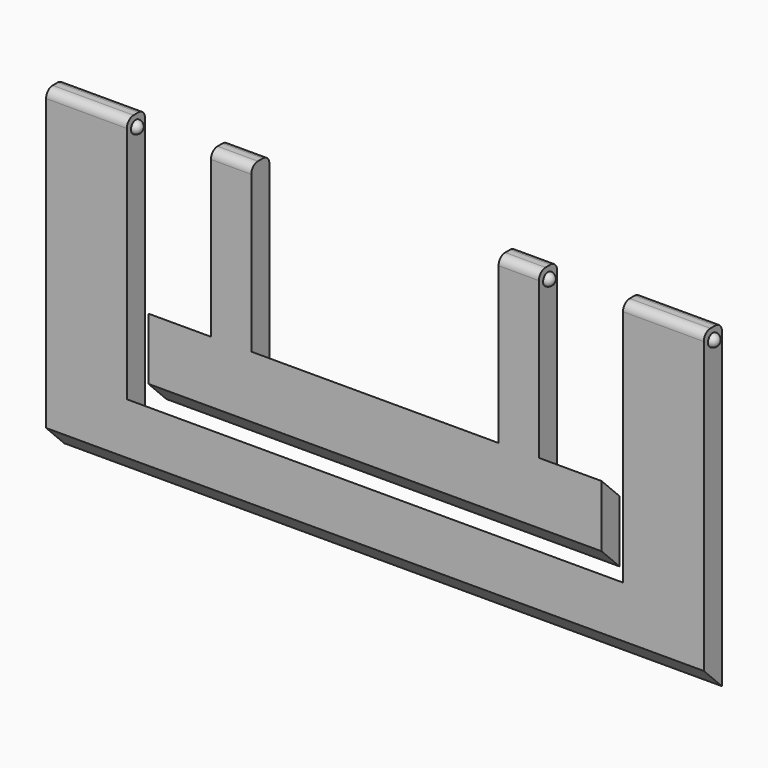
from build123d import *

# Parameters (mm, degrees)
F1_DEPTH       = 79.8
F1_DEPTH_BACK  = 79.8
F2_DEPTH       = 60.2
F2_DEPTH_BACK  = 60.2
F3_DEPTH       = 55
F3_DEPTH_BACK  = 55
F4_DEPTH       = 39.8
F4_DEPTH_BACK  = 39.8
F5_DEPTH       = 20.2
F5_DEPTH_BACK  = 20.2
F6_R           = 1.5
F7_DEPTH       = 1.5
F7_DEPTH_BACK  = 21.1
F8_R           = 1.49999
F9_R           = 1.5
F10_DEPTH      = 1.5
F10_DEPTH_BACK = 21.1
F11_R          = 1.49999
F12_R          = 1.5
F13_DEPTH      = 1.5
F13_DEPTH_BACK = 21.1
F14_R          = 1.49999
F15_R          = 1.5
F16_DEPTH      = 1.5
F16_DEPTH_BACK = 21.1
F17_R          = 1.49999
F18_DEPTH      = 30
F18_DEPTH_BACK = 30


# Not quite as in the source:
# - a fillet or chamfer is up to 0.001 mm smaller than in the source, because OpenCascade refuses the exact size


with BuildPart() as f1:
    # F0 (on Right) → F1 (new body, two sides)
    with BuildSketch(Plane.YZ) as f1_sk:
        with BuildLine():
            Line((-5.401472277, 44.6310500277), (-5.401472277, 79.9993566108))
            Line((-5.401472277, 79.9993566108), (-5.401472277, 88))
            ThreePointArc((-5.401472277, 88), (-5.9872587146, 89.4142135624), (-7.401472277, 90))
            Line((-7.401472277, 90), (-8.901472277, 90))
            ThreePointArc((-8.901472277, 90), (-10.3156858394, 89.4142135624), (-10.901472277, 88))
            Line((-10.901472277, 88), (-10.901472277, 80))
            Line((-10.901472277, 80), (-10.901472277, 50.1310500277))
            Line((-10.901472277, 50.1310500277), (-5.401472277, 44.6310500277))
        make_face()
        Polygon((-5.401472277, 29.6310500277), (-5.401472277, 44.6310500277), (-10.901472277, 50.1310500277), (-10.901472277, 35.1310500277), align=None)
        Polygon((-5.401472277, 24.6310500277), (-5.401472277, 29.6310500277), (-10.901472277, 35.1310500277), (-10.901472277, 30.1310500277), align=None)
        Polygon((-5.401472277, 18.0382234147), (-5.401472277, 24.6310500277), (-10.901472277, 30.1310500277), (-10.901472277, 17.6310500277), (-5.401472277, 12.1310500277), align=None)
    extrude(amount=F1_DEPTH)
    extrude(f1_sk.sketch, amount=-F1_DEPTH_BACK)

    # F0 (on Right) → F2 (cut, two sides)
    with BuildSketch(Plane.YZ) as f2_sk:
        Polygon((-5.401472277, 24.6310500277), (-5.401472277, 29.6310500277), (-10.901472277, 35.1310500277), (-10.901472277, 30.1310500277), align=None)
        Polygon((-5.401472277, 29.6310500277), (-5.401472277, 44.6310500277), (-10.901472277, 50.1310500277), (-10.901472277, 35.1310500277), align=None)
        with BuildLine():
            Line((-5.401472277, 44.6310500277), (-5.401472277, 79.9993566108))
            Line((-5.401472277, 79.9993566108), (-5.401472277, 88))
            ThreePointArc((-5.401472277, 88), (-5.9872587146, 89.4142135624), (-7.401472277, 90))
            Line((-7.401472277, 90), (-8.901472277, 90))
            ThreePointArc((-8.901472277, 90), (-10.3156858394, 89.4142135624), (-10.901472277, 88))
            Line((-10.901472277, 88), (-10.901472277, 80))
            Line((-10.901472277, 80), (-10.901472277, 50.1310500277))
            Line((-10.901472277, 50.1310500277), (-5.401472277, 44.6310500277))
        make_face()
    extrude(amount=F2_DEPTH, mode=Mode.SUBTRACT)
    extrude(f2_sk.sketch, amount=-F2_DEPTH_BACK, mode=Mode.SUBTRACT)

    # F6 (on face) → F7 (join, two sides)
    with BuildSketch(Plane(origin=(-79.8, 0, 0), x_dir=(0, -1, 0), z_dir=(-1, 0, 0))) as f7_sk:
        with Locations((8.151472277, 87.25)):
            Circle(F6_R)
    extrude(amount=F7_DEPTH)
    extrude(f7_sk.sketch, amount=-F7_DEPTH_BACK)

    # F8 (radius 1.5 in the source; OpenCascade refuses exactly that, so slightly less here)
    f8_edges = [f1.edges().sort_by_distance(p)[0] for p in [
        (-81.3, -6.651472, 87.25),
        (-58.7, -6.651472, 87.25),
    ]]
    fillet(f8_edges, radius=F8_R)

    # F15 (on face) → F16 (join, two sides)
    with BuildSketch(Plane(origin=(60.2, 0, 0), x_dir=(0, -1, 0), z_dir=(-1, 0, 0))) as f16_sk:
        with Locations((8.151472277, 87.25)):
            Circle(F15_R)
    extrude(amount=F16_DEPTH)
    extrude(f16_sk.sketch, amount=-F16_DEPTH_BACK)

    # F17 (radius 1.5 in the source; OpenCascade refuses exactly that, so slightly less here)
    f17_edges = [f1.edges().sort_by_distance(p)[0] for p in [
        (58.7, -6.651472, 87.25),
        (81.3, -6.651472, 87.25),
    ]]
    fillet(f17_edges, radius=F17_R)


with BuildPart() as f3:
    # F0 (on Right) → F3 (new body, two sides)
    with BuildSketch(Plane.YZ) as f3_sk:
        Polygon((-5.401472277, 29.6310500277), (-5.401472277, 44.6310500277), (-10.901472277, 50.1310500277), (-10.901472277, 35.1310500277), align=None)
    extrude(amount=F3_DEPTH)
    extrude(f3_sk.sketch, amount=-F3_DEPTH_BACK)

    # F0 (on Right) → F4 (join, two sides)
    with BuildSketch(Plane.YZ) as f4_sk:
        with BuildLine():
            Line((-5.401472277, 44.6310500277), (-5.401472277, 79.9993566108))
            Line((-5.401472277, 79.9993566108), (-5.401472277, 88))
            ThreePointArc((-5.401472277, 88), (-5.9872587146, 89.4142135624), (-7.401472277, 90))
            Line((-7.401472277, 90), (-8.901472277, 90))
            ThreePointArc((-8.901472277, 90), (-10.3156858394, 89.4142135624), (-10.901472277, 88))
            Line((-10.901472277, 88), (-10.901472277, 80))
            Line((-10.901472277, 80), (-10.901472277, 50.1310500277))
            Line((-10.901472277, 50.1310500277), (-5.401472277, 44.6310500277))
        make_face()
    extrude(amount=F4_DEPTH)
    extrude(f4_sk.sketch, amount=-F4_DEPTH_BACK)

    # F0 (on Right) → F5 (cut, two sides)
    with BuildSketch(Plane.YZ) as f5_sk:
        with BuildLine():
            Line((-5.401472277, 44.6310500277), (-5.401472277, 79.9993566108))
            Line((-5.401472277, 79.9993566108), (-5.401472277, 88))
            ThreePointArc((-5.401472277, 88), (-5.9872587146, 89.4142135624), (-7.401472277, 90))
            Line((-7.401472277, 90), (-8.901472277, 90))
            ThreePointArc((-8.901472277, 90), (-10.3156858394, 89.4142135624), (-10.901472277, 88))
            Line((-10.901472277, 88), (-10.901472277, 80))
            Line((-10.901472277, 80), (-10.901472277, 50.1310500277))
            Line((-10.901472277, 50.1310500277), (-5.401472277, 44.6310500277))
        make_face()
    extrude(amount=F5_DEPTH, mode=Mode.SUBTRACT)
    extrude(f5_sk.sketch, amount=-F5_DEPTH_BACK, mode=Mode.SUBTRACT)

    # F9 (on face) → F10 (join, two sides)
    with BuildSketch(Plane(origin=(-39.8, 0, 0), x_dir=(0, -1, 0), z_dir=(-1, 0, 0))) as f10_sk:
        with Locations((8.151472277, 87.25)):
            Circle(F9_R)
    extrude(amount=F10_DEPTH)
    extrude(f10_sk.sketch, amount=-F10_DEPTH_BACK)

    # F11 (radius 1.5 in the source; OpenCascade refuses exactly that, so slightly less here)
    f11_edges = [f3.edges().sort_by_distance(p)[0] for p in [
        (-41.3, -6.651472, 87.25),
        (-18.7, -6.651472, 87.25),
    ]]
    fillet(f11_edges, radius=F11_R)

    # F12 (on face) → F13 (join, two sides)
    with BuildSketch(Plane(origin=(20.2, 0, 0), x_dir=(0, -1, 0), z_dir=(-1, 0, 0))) as f13_sk:
        with Locations((8.151472277, 87.25)):
            Circle(F12_R)
    extrude(amount=F13_DEPTH)
    extrude(f13_sk.sketch, amount=-F13_DEPTH_BACK)

    # F14 (radius 1.5 in the source; OpenCascade refuses exactly that, so slightly less here)
    f14_edges = [f3.edges().sort_by_distance(p)[0] for p in [
        (18.7, -6.651472, 87.25),
        (41.3, -6.651472, 87.25),
    ]]
    fillet(f14_edges, radius=F14_R)

    # F0 (on Right) → F18 (cut, two sides)
    with BuildSketch(Plane.YZ) as f18_sk:
        with BuildLine():
            Line((-5.401472277, 44.6310500277), (-5.401472277, 79.9993566108))
            Line((-5.401472277, 79.9993566108), (-5.401472277, 88))
            ThreePointArc((-5.401472277, 88), (-5.9872587146, 89.4142135624), (-7.401472277, 90))
            Line((-7.401472277, 90), (-8.901472277, 90))
            ThreePointArc((-8.901472277, 90), (-10.3156858394, 89.4142135624), (-10.901472277, 88))
            Line((-10.901472277, 88), (-10.901472277, 80))
            Line((-10.901472277, 80), (-10.901472277, 50.1310500277))
            Line((-10.901472277, 50.1310500277), (-5.401472277, 44.6310500277))
        make_face()
    extrude(amount=-F18_DEPTH, mode=Mode.SUBTRACT)
    extrude(f18_sk.sketch, amount=F18_DEPTH_BACK, mode=Mode.SUBTRACT)


solid = Compound([f1.part, f3.part])
